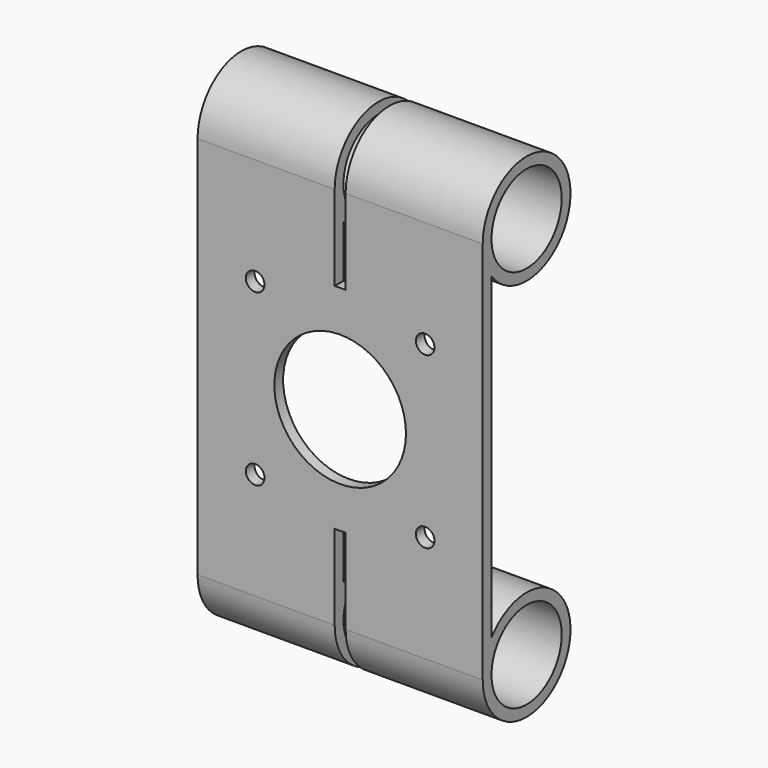
from build123d import *

# Parameters (mm, degrees)
F0_R     = 8
F1_DEPTH = 26
F2_R     = 12
F2_R_2   = 1.7
F3_DEPTH = 25
F5_DEPTH = 20.001


# Not quite as in the source:
# - a pattern or mirror of a feature is missing from the dataset's text; its kind, count and spacing are read off the source's solid


with BuildPart() as f1:
    # F0 (on Right) → F1 (new body, symmetric)
    with BuildSketch(Plane.YZ):
        with BuildLine():
            ThreePointArc((2, 29), (19.4868329805, 38.1622776602), (0, 35))
            Line((0, 35), (0, -35))
            ThreePointArc((0, -35), (19.4868329805, -38.1622776602), (2, -29))
            Line((2, -29), (2, 29))
        make_face()
        with Locations((10, -35)):
            Circle(F0_R, mode=Mode.SUBTRACT)
        with Locations((10, 35)):
            Circle(F0_R, mode=Mode.SUBTRACT)
    extrude(amount=F1_DEPTH, both=True)

    # F2 (on face) → F3 (cut)
    with BuildSketch(Plane.XZ):
        Circle(F2_R)
        with Locations((-15.5, 15.5)):
            Circle(F2_R_2)
        with Locations((15.5, 15.5)):
            Circle(F2_R_2)
        with Locations((15.5, -15.5)):
            Circle(F2_R_2)
        with Locations((-15.5, -15.5)):
            Circle(F2_R_2)
    extrude(amount=-F3_DEPTH, mode=Mode.SUBTRACT)

    # F4 (on face) → F5 (cut, through all)
    with BuildSketch(Plane.XZ):
        with BuildLine():
            Line((1, 19.4743420942), (1, 45))
            Line((1, 45), (-1, 45))
            Line((-1, 45), (-1, 19.4743420942))
            ThreePointArc((-1, 19.4743420942), (0, 19.5), (1, 19.4743420942))
        make_face()
    f5 = extrude(amount=-F5_DEPTH, mode=Mode.SUBTRACT)

    # F5_copies: F5 across plane
    add(f5.mirror(Plane(origin=(0, 0, 0), x_dir=(-1, 0, 0), z_dir=(0, 0, -1))), mode=Mode.SUBTRACT)


solid = f1.part
